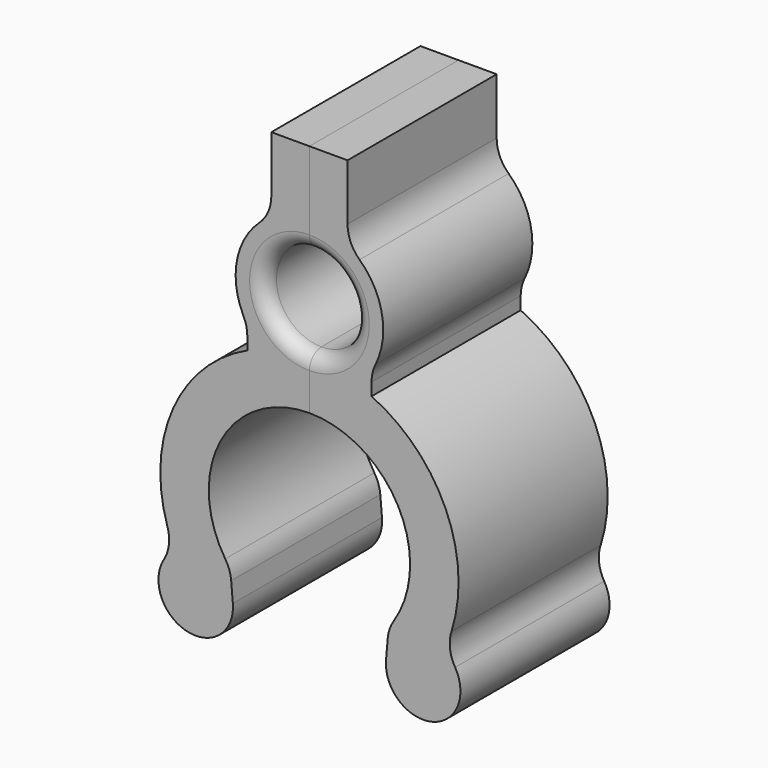
from build123d import *

# Parameters (mm, degrees)
F1_DEPTH = 25
F3_R     = 5
F3_2_R   = 5
F4_R     = 2
F4_2_R   = 2


with BuildPart() as f1:
    # F0 (on Front) → F1 (new body)
    with BuildSketch(Plane.XZ):
        with BuildLine():
            ThreePointArc((0, -13.0244963626), (12.1428481509, -20.6252388852), (10.6124130002, -34.8687572833))
            Line((10.6124130002, -34.8687572833), (10.2718717194, -38.8542348753))
            ThreePointArc((10.2718717194, -38.8542348753), (17.410017551, -43.7910505016), (18.0512113015, -35.1357547229))
            ThreePointArc((18.0512113015, -35.1357547229), (18.8012077702, -19.7043360726), (8.3319982441, -8.3426976271))
            Line((8.3319982441, -8.3426976271), (8.3319982441, -5.3426976271))
            ThreePointArc((8.3319982441, -5.3426976271), (9.6395478341, 2.246270293), (5.111990881, 8.4755036374))
            Line((5.111990881, 8.4755036374), (5.111990881, 18.4755036374))
            Line((5.111990881, 18.4755036374), (0, 18.4755036374))
            Line((0, 18.4755036374), (0, 6.0244963626))
            ThreePointArc((0, 6.0244963626), (6.0244963626, 0), (0, -6.0244963626))
            Line((0, -6.0244963626), (0, -13.0244963626))
        make_face()
    extrude(amount=F1_DEPTH)


with BuildPart() as f2_1:
    # F2: instance of F1
    add(f1.part.mirror(Plane.YZ))

    # F3#2
    f3_2_edges = [f2_1.edges().sort_by_distance(p)[0] for p in [
        (-10.612413, -12.5, -34.868757),
        (-18.051211, -12.5, -35.135755),
        (-5.111991, -12.5, 8.475504),
        (-8.331998, -12.5, -5.342698),
    ]]
    fillet(f3_2_edges, radius=F3_2_R)

    # F4#2
    f4_2_edges = [f2_1.edges().sort_by_distance(p)[0] for p in [
        (-6.024496, -25, 0),
        (-6.024496, 0, 0),
    ]]
    fillet(f4_2_edges, radius=F4_2_R)


with BuildPart() as f1_1:
    add(f1.part)

    # F3
    f3_edges = [f1_1.edges().sort_by_distance(p)[0] for p in [
        (10.612413, -12.5, -34.868757),
        (18.051211, -12.5, -35.135755),
        (5.111991, -12.5, 8.475504),
        (8.331998, -12.5, -5.342698),
    ]]
    fillet(f3_edges, radius=F3_R)

    # F4
    f4_edges = [f1_1.edges().sort_by_distance(p)[0] for p in [
        (6.024496, -25, 0),
        (6.024496, 0, 0),
    ]]
    fillet(f4_edges, radius=F4_R)


solid = Compound([f2_1.part, f1_1.part])
